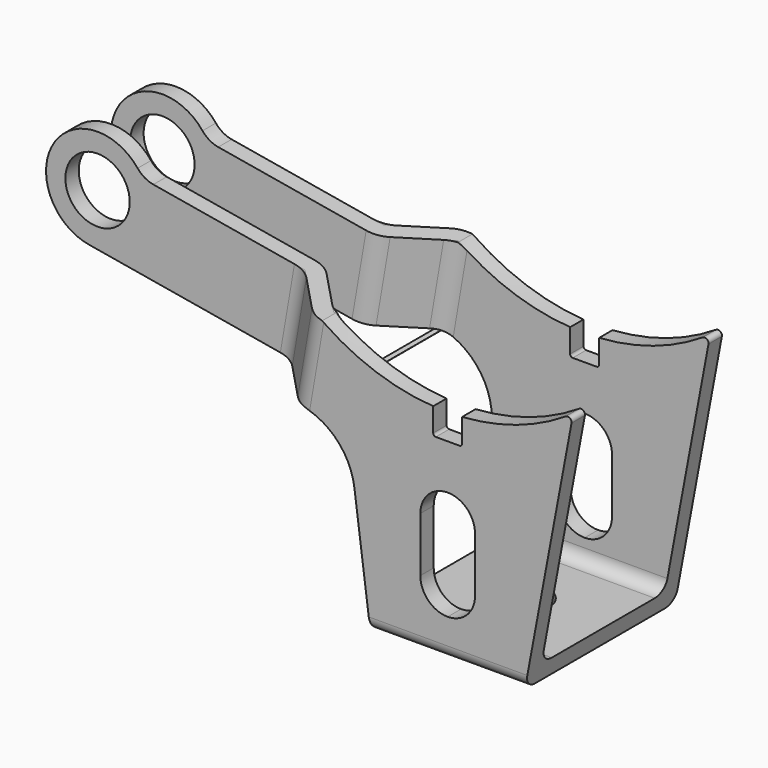
from build123d import *

# Parameters (mm, degrees)
F1_DEPTH       = 7.3
F1_DEPTH_BACK  = 7.3
F3_DEPTH       = 6
F3_DEPTH_BACK  = 6
F5_DEPTH       = 10
F5_DEPTH_BACK  = 10
F8_DEPTH       = 25
F9_R           = 2.5
F10_DEPTH      = 10
F10_DEPTH_BACK = 10
F11_T1_DEPTH   = 6.5
F11_T6_DEPTH   = 12.7132034356
F11_S7_R       = 5
F11_T8_DEPTH   = 8
F11_S10_R      = 17
F11_T11_DEPTH  = 8
F11_T15_DEPTH  = 8.5710678119
F11_T20_DEPTH  = 12.7132034356
F11_S21_R      = 5
F11_T22_DEPTH  = 8
F11_S24_R      = 17
F11_T25_DEPTH  = 8
F11_T29_DEPTH  = 8.5710678119
F11_T31_DEPTH  = 10.6421356237
F12_R          = 1
F13_R          = 2
F14_DEPTH      = 5


# Not quite as in the source:
# - a fillet or chamfer that OpenCascade refuses, or shapes differently, is made with other operations: its cross-section is extruded or revolved along the edge and cut away or added


with BuildPart() as f1:
    # F0 (on Front) → F1 (new body, two sides)
    with BuildSketch(Plane.XZ) as f1_sk:
        with BuildLine():
            Line((-7.2480415045, 9.479816391), (-6, 0))
            Line((-6, 0), (6, 0))
            Line((6, 0), (9.6197658273, 19.3731186918))
            ThreePointArc((9.6197658273, 19.3731186918), (9.492555749, 19.6769779623), (9.1631662961, 19.6809084286))
            ThreePointArc((9.1631662961, 19.6809084286), (-0.3536100614, 17.0036780472), (-9.750799418, 20.0744152471))
            Line((-9.750799418, 20.0744152471), (-25.666835692, 22.7954629152))
            ThreePointArc((-25.666835692, 22.7954629152), (-26.3420622378, 23.0419468668), (-26.8865335991, 23.511240126))
            ThreePointArc((-26.8865335991, 23.511240126), (-33.4498266444, 23.0245236782), (-30.6740705867, 17.0572054525))
            Line((-30.6740705867, 17.0572054525), (-11.362677578, 13.7556786143))
            ThreePointArc((-11.362677578, 13.7556786143), (-8.6024605414, 12.2941429125), (-7.2480415045, 9.479816391))
        make_face()
    extrude(amount=F1_DEPTH)
    extrude(f1_sk.sketch, amount=-F1_DEPTH_BACK)

    # F2 (on Front) → F3 (cut, two sides)
    with BuildSketch(Plane.XZ) as f3_sk:
        Polygon((15, 1.3), (15, 78.0352148958), (0, 78.0352148958), (-11, 13.6936742961), (-11, 1.3), align=None)
    extrude(amount=F3_DEPTH, mode=Mode.SUBTRACT)
    extrude(f3_sk.sketch, amount=-F3_DEPTH_BACK, mode=Mode.SUBTRACT)

    # F4 (on Front) → F5 (cut, two sides)
    with BuildSketch(Plane.XZ) as f5_sk:
        with BuildLine():
            Line((0, 18), (-1.125, 18))
            Line((-1.125, 18), (-1.125, 15.2))
            ThreePointArc((-1.125, 15.2), (-1.0664213562, 15.0585786438), (-0.925, 15))
            Line((-0.925, 15), (0, 15))
            Line((0, 15), (0.925, 15))
            ThreePointArc((0.925, 15), (1.0664213562, 15.0585786438), (1.125, 15.2))
            Line((1.125, 15.2), (1.125, 18))
            Line((1.125, 18), (0, 18))
        make_face()
        with BuildLine():
            ThreePointArc((0, 11.5), (-1.50260191, 10.87760191), (-2.125, 9.375))
            Line((-2.125, 9.375), (-2.125, 5.125))
            ThreePointArc((-2.125, 5.125), (-1.50260191, 3.62239809), (0, 3))
            ThreePointArc((0, 3), (1.50260191, 3.62239809), (2.125, 5.125))
            Line((2.125, 5.125), (2.125, 9.375))
            ThreePointArc((2.125, 9.375), (1.50260191, 10.87760191), (0, 11.5))
        make_face()
    extrude(amount=F5_DEPTH, mode=Mode.SUBTRACT)
    extrude(f5_sk.sketch, amount=-F5_DEPTH_BACK, mode=Mode.SUBTRACT)

    # F7 (on offset) → F8 (cut)
    with BuildSketch(Plane(origin=(1.9622434031, 0, 11.4776148716), x_dir=(0.9856986369, 0, -0.1685176467), z_dir=(-0.1685176467, 0, -0.9856986369))):
        Polygon((-41.9907133171, -7.3), (-13.6887884036, -7.3), (-17.1887884036, -3.8), (-41.9907133171, -3.8), align=None)
        Polygon((-41.9907133171, 7.3), (-41.9907133171, 3.8), (-17.1887884036, 3.8), (-13.6887884036, 7.3), align=None)
        Polygon((-16.6503107725, -2.5), (-13.1503107725, -6), (-13.1503107725, 0), (-13.1503107725, 6), (-16.6503107725, 2.5), (-41.9907133171, 2.5), (-41.9907133171, 0), (-41.9907133171, -2.5), align=None)
    extrude(amount=-F8_DEPTH, mode=Mode.SUBTRACT)

    # F9 (on Front) → F10 (cut, two sides)
    with BuildSketch(Plane.XZ) as f10_sk:
        with Locations((-30, 21)):
            Circle(F9_R)
    extrude(amount=F10_DEPTH, mode=Mode.SUBTRACT)
    extrude(f10_sk.sketch, amount=-F10_DEPTH_BACK, mode=Mode.SUBTRACT)

    # F11: fillet of radius 2 on 8 edges, made by hand

    # F11_s2 → F11_t1 (join)
    with BuildSketch(Plane(origin=(1.9622434031, 0, 11.4776148716), x_dir=(0, 1, 0), z_dir=(0.1685176467, 0, 0.9856986369))):
        with BuildLine():
            ThreePointArc((3.8, 18.0172155284), (3.952240935, 17.2518486636), (4.3857864376, 16.603001966))
            Line((4.3857864376, 16.603001966), (3.8, 17.1887884036))
            Line((3.8, 17.1887884036), (3.8, 18.0172155284))
        make_face()
        with BuildLine():
            ThreePointArc((-4.3857864376, 16.603001966), (-3.952240935, 17.2518486636), (-3.8, 18.0172155284))
            Line((-3.8, 18.0172155284), (-3.8, 17.1887884036))
            Line((-3.8, 17.1887884036), (-4.3857864376, 16.603001966))
        make_face()
    extrude(amount=F11_T1_DEPTH)


with BuildPart() as f11_tool4:
    # F11_s5 → F11_t6 (new body)
    with BuildSketch(Plane(origin=(3.0576081065, 0, 17.8846560114), x_dir=(0, 1, 0), z_dir=(-0.1685176467, 0, -0.9856986369))):
        with BuildLine():
            ThreePointArc((-6, -12.3218836478), (-5.847759065, -13.0872505125), (-5.4142135624, -13.7360972102))
            Line((-5.4142135624, -13.7360972102), (-6, -13.1503107725))
            Line((-6, -13.1503107725), (-6, -12.3218836478))
        make_face()
    extrude(amount=F11_T6_DEPTH)

    # F11_s7 → F11_t8 (cut, symmetric)
    with BuildSketch(Plane.XZ.offset(5.7)):
        with Locations((-12.2052658114, 8.8271854299)):
            Circle(F11_S7_R)
    extrude(amount=F11_T8_DEPTH, both=True, mode=Mode.SUBTRACT)

    split(bisect_by=Plane.YZ.offset(-11), keep=Keep.TOP)

    # F11_s10 → F11_t11 (cut, symmetric)
    with BuildSketch(Plane.XZ.offset(5.7)):
        with Locations((0, 34)):
            Circle(F11_S10_R)
    extrude(amount=F11_T11_DEPTH, both=True, mode=Mode.SUBTRACT)


with BuildPart() as f1_1:
    add(f1.part)

    # F11_t3: union F11_tool4
    add(f11_tool4.part)


with BuildPart() as f11_tool13:
    # F11_s14 → F11_t15 (new body)
    with BuildSketch(Plane(origin=(3.4066195803, 0, 19.9261047304), x_dir=(0, 1, 0), z_dir=(-0.1685176467, 0, -0.9856986369))):
        with BuildLine():
            ThreePointArc((-6, -12.3218836478), (-5.847759065, -13.0872505125), (-5.4142135624, -13.7360972102))
            Line((-5.4142135624, -13.7360972102), (-6, -13.1503107725))
            Line((-6, -13.1503107725), (-6, -12.3218836478))
        make_face()
    extrude(amount=F11_T15_DEPTH)

    split(bisect_by=Plane.YZ.offset(-11), keep=Keep.BOTTOM)


with BuildPart() as f1_2:
    add(f1_1.part)

    # F11_t12: union F11_tool13
    add(f11_tool13.part)


with BuildPart() as f11_tool18:
    # F11_s19 → F11_t20 (new body)
    with BuildSketch(Plane(origin=(3.0576081065, 0, 17.8846560114), x_dir=(0, 1, 0), z_dir=(-0.1685176467, 0, -0.9856986369))):
        with BuildLine():
            ThreePointArc((6, -12.3218836478), (5.847759065, -13.0872505125), (5.4142135624, -13.7360972102))
            Line((5.4142135624, -13.7360972102), (6, -13.1503107725))
            Line((6, -13.1503107725), (6, -12.3218836478))
        make_face()
    extrude(amount=F11_T20_DEPTH)

    # F11_s21 → F11_t22 (cut, symmetric)
    with BuildSketch(Plane.XZ.offset(-5.7)):
        with Locations((-12.2052658114, 8.8271854299)):
            Circle(F11_S21_R)
    extrude(amount=F11_T22_DEPTH, both=True, mode=Mode.SUBTRACT)

    split(bisect_by=Plane.YZ.offset(-11), keep=Keep.TOP)

    # F11_s24 → F11_t25 (cut, symmetric)
    with BuildSketch(Plane.XZ.offset(-5.7)):
        with Locations((0, 34)):
            Circle(F11_S24_R)
    extrude(amount=F11_T25_DEPTH, both=True, mode=Mode.SUBTRACT)


with BuildPart() as f1_3:
    add(f1_2.part)

    # F11_t17: union F11_tool18
    add(f11_tool18.part)


with BuildPart() as f11_tool27:
    # F11_s28 → F11_t29 (new body)
    with BuildSketch(Plane(origin=(3.4066195803, 0, 19.9261047304), x_dir=(0, 1, 0), z_dir=(-0.1685176467, 0, -0.9856986369))):
        with BuildLine():
            ThreePointArc((6, -12.3218836478), (5.847759065, -13.0872505125), (5.4142135624, -13.7360972102))
            Line((5.4142135624, -13.7360972102), (6, -13.1503107725))
            Line((6, -13.1503107725), (6, -12.3218836478))
        make_face()
    extrude(amount=F11_T29_DEPTH)

    split(bisect_by=Plane.YZ.offset(-11), keep=Keep.BOTTOM)


with BuildPart() as f1_4:
    add(f1_3.part)

    # F11_t26: union F11_tool27
    add(f11_tool27.part)

    # F11_s32 → F11_t31 (cut)
    with BuildSketch(Plane(origin=(1.6132319293, 0, 9.4361661525), x_dir=(0, 1, 0), z_dir=(0.1685176467, 0, 0.9856986369))):
        with BuildLine():
            ThreePointArc((6.7142135624, 14.2745748413), (7.147759065, 13.6257281436), (7.3, 12.8603612789))
            Line((7.3, 12.8603612789), (7.3, 13.6887884036))
            Line((7.3, 13.6887884036), (6.7142135624, 14.2745748413))
        make_face()
        with BuildLine():
            ThreePointArc((-2.5, 17.4787378973), (-2.652240935, 16.7133710326), (-3.0857864376, 16.0645243349))
            Line((-3.0857864376, 16.0645243349), (-2.5, 16.6503107725))
            Line((-2.5, 16.6503107725), (-2.5, 17.4787378973))
        make_face()
        with BuildLine():
            ThreePointArc((-6.7142135624, 14.2745748413), (-7.147759065, 13.6257281436), (-7.3, 12.8603612789))
            Line((-7.3, 12.8603612789), (-7.3, 13.6887884036))
            Line((-7.3, 13.6887884036), (-6.7142135624, 14.2745748413))
        make_face()
        with BuildLine():
            ThreePointArc((2.5, 17.4787378973), (2.652240935, 16.7133710326), (3.0857864376, 16.0645243349))
            Line((3.0857864376, 16.0645243349), (2.5, 16.6503107725))
            Line((2.5, 16.6503107725), (2.5, 17.4787378973))
        make_face()
    extrude(amount=F11_T31_DEPTH, mode=Mode.SUBTRACT)

    # F12
    f12_edges = [f1_4.edges().sort_by_distance(p)[0] for p in [
        (0.035875, 6, 1.3),
        (0, -7.3, 0),
        (0.035875, -6, 1.3),
        (0, 7.3, 0),
    ]]
    fillet(f12_edges, radius=F12_R)

    # F13 (on Top) → F14 (cut)
    with BuildSketch(Plane.XY):
        Circle(F13_R)
    extrude(amount=F14_DEPTH, mode=Mode.SUBTRACT)


solid = f1_4.part
